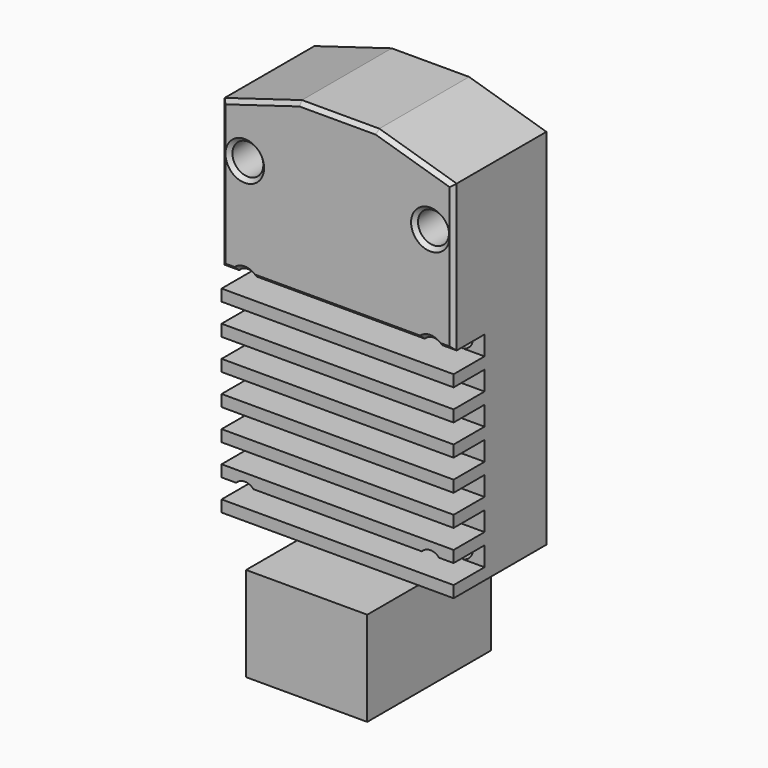
from build123d import *

# Parameters (mm, degrees)
F0_R       = 1.5
F0_R_2     = 2
F1_DEPTH   = 15
F2_W       = 5
F2_H       = 2.5
F3_DEPTH   = 30.001
F5_SIZE2   = 10
F5_SIZE    = 3
F5_2_SIZE2 = 10
F5_2_SIZE  = 3
F6_SIZE    = 0.49999
F4_R       = 3
F7_DEPTH   = 19.5
F8_SIZE    = 3
F9_W       = 15.6673565507
F9_H       = 12.20472157
F10_DEPTH  = 20


# Not quite as in the source:
# - a fillet or chamfer is up to 0.001 mm smaller than in the source, because OpenCascade refuses the exact size


with BuildPart() as f1:
    # F0 (on Front) → F1 (new body)
    with BuildSketch(Plane.XZ):
        Polygon((15, 0), (0, 0), (-15, 0), (-15, -50), (0, -50), (15, -50), align=None)
        with Locations((-12, -47)):
            Circle(F0_R, mode=Mode.SUBTRACT)
        with Locations((12, -47)):
            Circle(F0_R, mode=Mode.SUBTRACT)
        with Locations((-12, -23)):
            Circle(F0_R, mode=Mode.SUBTRACT)
        with Locations((-12, -9)):
            Circle(F0_R_2, mode=Mode.SUBTRACT)
        with Locations((12, -23)):
            Circle(F0_R, mode=Mode.SUBTRACT)
        with Locations((12, -9)):
            Circle(F0_R_2, mode=Mode.SUBTRACT)
    extrude(amount=F1_DEPTH)

    # F2 (on face) → F3 (cut, through all)
    with BuildSketch(Plane(origin=(-15, 0, 0), x_dir=(0, -1, 0), z_dir=(-1, 0, 0))):
        with Locations((12.5, -47.25)):
            Rectangle(F2_W, F2_H)
        with Locations((12.5, -43.25)):
            Rectangle(F2_W, F2_H)
        with Locations((12.5, -39.25)):
            Rectangle(F2_W, F2_H)
        with Locations((12.5, -35.25)):
            Rectangle(F2_W, F2_H)
        with Locations((12.5, -31.25)):
            Rectangle(F2_W, F2_H)
        with Locations((12.5, -27.25)):
            Rectangle(F2_W, F2_H)
        with Locations((12.5, -23.25)):
            Rectangle(F2_W, F2_H)
    extrude(amount=-F3_DEPTH, mode=Mode.SUBTRACT)

    # F5
    f5_edges = [f1.edges().sort_by_distance(p)[0] for p in [
        (-15, -7.5, 0),
    ]]
    f5_side = f1.faces().sort_by_distance((-15, -6.839623, -23.646226))[0]
    chamfer(f5_edges, length=F5_SIZE, length2=F5_SIZE2, reference=f5_side)

    # F5#2
    f5_2_edges = [f1.edges().sort_by_distance(p)[0] for p in [
        (15, -7.5, 0),
    ]]
    f5_2_side = f1.faces().sort_by_distance((15, -6.839623, -23.646226))[0]
    chamfer(f5_2_edges, length=F5_2_SIZE, length2=F5_2_SIZE2, reference=f5_2_side)

    # F6 (size 0.5 in the source; OpenCascade refuses exactly that, so slightly less here)
    f6_edges = [f1.edges().sort_by_distance(p)[0] for p in [
        (0, -15, 0),
        (10, -15, -1.5),
        (-10, -15, -1.5),
        (15, -15, -12.5),
        (-15, -15, -12.5),
        (14.059017, -15, -22),
        (-14.059017, -15, -22),
        (12, -15, -21.5),
        (-12, -15, -21.5),
        (0, -15, -22),
        (-14, -15, -9),
        (10, -15, -9),
    ]]
    chamfer(f6_edges, length=F6_SIZE)

    # F4 (on face) → F7 (join)
    with BuildSketch(Plane(origin=(0, 0, -50), x_dir=(1, 0, 0), z_dir=(0, 0, -1))):
        with Locations((0, 5)):
            Circle(F4_R)
    extrude(amount=F7_DEPTH)

    # F8
    f8_edges = [f1.edges().sort_by_distance(p)[0] for p in [
        (-3, -5, -69.5),
    ]]
    chamfer(f8_edges, length=F8_SIZE)

    # F9 (on Front) → F10 (join)
    with BuildSketch(Plane.XZ):
        with Locations((0, -58.2721680403)):
            Rectangle(F9_W, F9_H)
    extrude(amount=F10_DEPTH)


solid = f1.part
